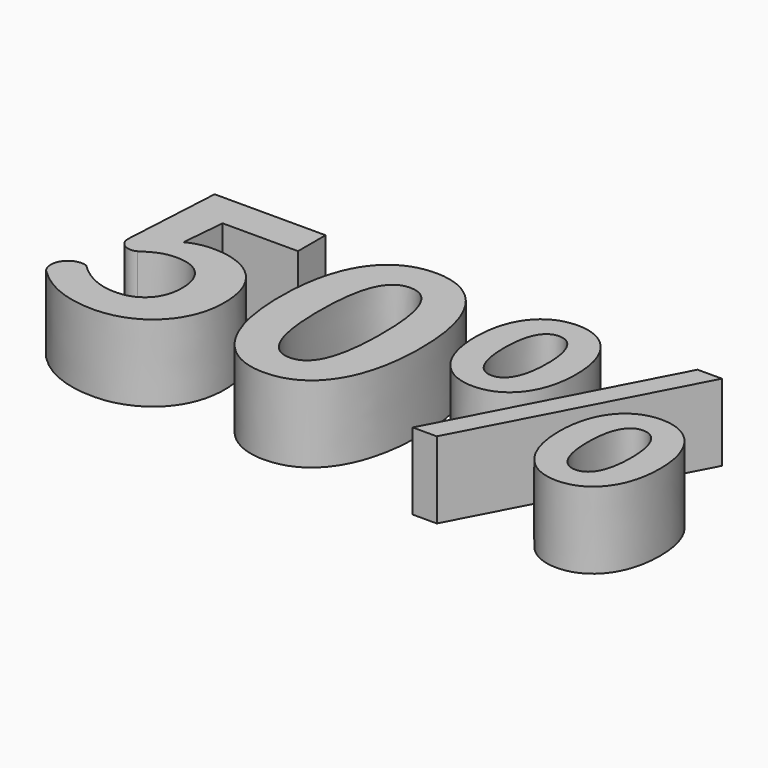
from build123d import *

# Parameters (mm, degrees)
F2_DEPTH = 40


with BuildPart() as f2:
    # F1 (on Top) → F2 (new body)
    with BuildSketch(Plane.XY):
        with BuildLine():
            Line((-37.6012061267, 49.3926707034), (-95.4441113863, 49.3926707034))
            Line((-95.4441113863, 49.3926707034), (-98.3659313836, -3.0631289361))
            ThreePointArc((-98.3659313836, -3.0631289361), (-95.3198653418, -9.0950649064), (-88.5732690488, -9.477436899))
            add(Edge.make_bspline(
                [(-88.5732690488, -9.477436899), (-82.2959213983, -5.3914542465), (-78.780606714, -3.7935839355), (-72.3662987511, -3.7935839355)],
                knots=[0, 0, 0, 0, 1, 1, 1, 1], degree=3))
            add(Edge.make_bspline(
                [(-72.3662987511, -3.7935839355), (-61.4094737612, -3.7935839355), (-54.1049237678, -10.8013865853), (-54.1049237678, -23.3560818864)],
                knots=[0, 0, 0, 0, 1, 1, 1, 1], degree=3))
            add(Edge.make_bspline(
                [(-54.1049237678, -23.3560818864), (-54.1049237678, -36.0705642185), (-61.9801417294, -43.2381538994), (-73.2337140629, -43.2381538994)],
                knots=[0, 0, 0, 0, 1, 1, 1, 1], degree=3))
            add(Edge.make_bspline(
                [(-73.2337140629, -43.2381538994), (-83.3231237411, -43.2381538994), (-90.9244210779, -38.2619292165), (-97.0419816974, -32.2813289094)],
                knots=[0, 0, 0, 0, 1, 1, 1, 1], degree=3))
            ThreePointArc((-97.0419816974, -32.2813289094), (-107.0940288058, -35.4584640814), (-106.9944310633, -46.0001868657))
            add(Edge.make_bspline(
                [(-106.9944310633, -46.0001868657), (-98.9594260706, -54.0351918583), (-87.546066706, -60.7690738834), (-70.4716810966, -60.7690738834)],
                knots=[0, 0, 0, 0, 1, 1, 1, 1], degree=3))
            add(Edge.make_bspline(
                [(-70.4716810966, -60.7690738834), (-50.4526487712, -60.7690738834), (-32.6249814437, -46.8904288961), (-32.6249814437, -22.7854139181)],
                knots=[0, 0, 0, 0, 1, 1, 1, 1], degree=3))
            add(Edge.make_bspline(
                [(-32.6249814437, -22.7854139181), (-32.6249814437, 0.7489330916), (-47.8275761173, 11.5459710505), (-65.9291640695, 11.5459710505)],
                knots=[0, 0, 0, 0, 1, 1, 1, 1], degree=3))
            add(Edge.make_bspline(
                [(-65.9291640695, 11.5459710505), (-70.9053887525, 11.5459710505), (-74.6946240615, 10.5415954264), (-78.9403937451, 8.4871907408)],
                knots=[0, 0, 0, 0, 1, 1, 1, 1], degree=3))
            Line((-78.9403937451, 8.4871907408), (-76.8859890595, 31.4280430636))
            Line((-76.8859890595, 31.4280430636), (-37.6012061267, 31.4280430636))
            Line((-37.6012061267, 31.4280430636), (-37.6012061267, 49.3926707034))
        make_face()
    extrude(amount=F2_DEPTH)


with BuildPart() as f2b:
    # F1 (on Top) → F2, piece 2 (new body)
    with BuildSketch(Plane.XY):
        with BuildLine():
            add(Edge.make_bspline(
                [(54.8926581638, -4.2272915913), (54.8926581638, 33.0259133746), (40.2835581772, 51.4470753891), (18.3699081972, 51.4470753891)],
                knots=[0, 0, 0, 0, 1, 1, 1, 1], degree=3))
            add(Edge.make_bspline(
                [(18.3699081972, 51.4470753891), (-3.6807020952, 51.4470753891), (-18.2898020818, 33.1857004057), (-18.2898020818, -4.2272915913)],
                knots=[0, 0, 0, 0, 1, 1, 1, 1], degree=3))
            add(Edge.make_bspline(
                [(-18.2898020818, -4.2272915913), (-18.2898020818, -41.4804965573), (-3.6807020952, -60.7690738834), (18.3699081972, -60.7690738834)],
                knots=[0, 0, 0, 0, 1, 1, 1, 1], degree=3))
            add(Edge.make_bspline(
                [(18.3699081972, -60.7690738834), (40.2835581772, -60.7690738834), (54.8926581638, -41.4804965573), (54.8926581638, -4.2272915913)],
                knots=[0, 0, 0, 0, 1, 1, 1, 1], degree=3))
        make_face()
        with BuildLine():
            add(Edge.make_bspline(
                [(34.5768784949, -4.2272915913), (34.5768784949, -34.6096542198), (27.569075845, -43.9686088988), (18.3699081972, -43.9686088988)],
                knots=[0, 0, 0, 0, 1, 1, 1, 1], degree=3))
            add(Edge.make_bspline(
                [(18.3699081972, -43.9686088988), (9.0109535183, -43.9686088988), (2.0031508684, -34.6096542198), (2.0031508684, -4.2272915913)],
                knots=[0, 0, 0, 0, 1, 1, 1, 1], degree=3))
            add(Edge.make_bspline(
                [(2.0031508684, -4.2272915913), (2.0031508684, 26.0181107248), (9.0109535183, 34.7835707168), (18.3699081972, 34.7835707168)],
                knots=[0, 0, 0, 0, 1, 1, 1, 1], degree=3))
            add(Edge.make_bspline(
                [(18.3699081972, 34.7835707168), (27.569075845, 34.7835707168), (34.5768784949, 26.0181107248), (34.5768784949, -4.2272915913)],
                knots=[0, 0, 0, 0, 1, 1, 1, 1], degree=3))
        make_face(mode=Mode.SUBTRACT)
    extrude(amount=F2_DEPTH)


with BuildPart() as f2c:
    # F1 (on Top) → F2, piece 3 (new body)
    with BuildSketch(Plane.XY):
        with BuildLine():
            add(Edge.make_bspline(
                [(118.7389904492, 17.3896110452), (118.7389904492, 39.0293404004), (107.7821654593, 51.4470753891), (92.3056501609, 51.4470753891)],
                knots=[0, 0, 0, 0, 1, 1, 1, 1], degree=3))
            add(Edge.make_bspline(
                [(92.3056501609, 51.4470753891), (76.8063081438, 51.4470753891), (66.0092701849, 39.0293404004), (66.0092701849, 17.3896110452)],
                knots=[0, 0, 0, 0, 1, 1, 1, 1], degree=3))
            add(Edge.make_bspline(
                [(66.0092701849, 17.3896110452), (66.0092701849, -4.3642519037), (76.8063081438, -17.0787342358), (92.3056501609, -17.0787342358)],
                knots=[0, 0, 0, 0, 1, 1, 1, 1], degree=3))
            add(Edge.make_bspline(
                [(92.3056501609, -17.0787342358), (107.7821654593, -17.0787342358), (118.7389904492, -4.3642519037), (118.7389904492, 17.3896110452)],
                knots=[0, 0, 0, 0, 1, 1, 1, 1], degree=3))
        make_face()
        with BuildLine():
            add(Edge.make_bspline(
                [(103.5592224944, 17.3896110452), (103.5592224944, 1.479388091), (98.5829978114, -4.9577465907), (92.3056501609, -4.9577465907)],
                knots=[0, 0, 0, 0, 1, 1, 1, 1], degree=3))
            add(Edge.make_bspline(
                [(92.3056501609, -4.9577465907), (86.0283025104, -4.9577465907), (81.1890381398, 1.479388091), (81.1890381398, 17.3896110452)],
                knots=[0, 0, 0, 0, 1, 1, 1, 1], degree=3))
            add(Edge.make_bspline(
                [(81.1890381398, 17.3896110452), (81.1890381398, 33.3226607181), (86.0283025104, 39.3032610251), (92.3056501609, 39.3032610251)],
                knots=[0, 0, 0, 0, 1, 1, 1, 1], degree=3))
            add(Edge.make_bspline(
                [(92.3056501609, 39.3032610251), (98.5829978114, 39.3032610251), (103.5592224944, 33.3226607181), (103.5592224944, 17.3896110452)],
                knots=[0, 0, 0, 0, 1, 1, 1, 1], degree=3))
        make_face(mode=Mode.SUBTRACT)
    extrude(amount=F2_DEPTH)


with BuildPart() as f2d:
    # F1 (on Top) → F2, piece 4 (new body)
    with BuildSketch(Plane.XY):
        Polygon((167.3827280611, 51.4470753891), (154.6910724477, 51.4470753891), (95.9579251576, -60.7690738834), (108.5126204586, -60.7690738834), align=None)
    extrude(amount=F2_DEPTH)


with BuildPart() as f2e:
    # F1 (on Top) → F2, piece 5 (new body)
    with BuildSketch(Plane.XY):
        with BuildLine():
            add(Edge.make_bspline(
                [(170.8980427453, -60.7690738834), (186.2375977313, -60.7690738834), (197.3313830337, -47.8948045202), (197.3313830337, -26.2779018837)],
                knots=[0, 0, 0, 0, 1, 1, 1, 1], degree=3))
            add(Edge.make_bspline(
                [(197.3313830337, -26.2779018837), (197.3313830337, -4.5240389348), (186.2375977313, 7.8936960538), (170.8980427453, 7.8936960538)],
                knots=[0, 0, 0, 0, 1, 1, 1, 1], degree=3))
            add(Edge.make_bspline(
                [(170.8980427453, 7.8936960538), (155.5584877594, 7.8936960538), (144.6016627694, -4.5240389348), (144.6016627694, -26.2779018837)],
                knots=[0, 0, 0, 0, 1, 1, 1, 1], degree=3))
            add(Edge.make_bspline(
                [(144.6016627694, -26.2779018837), (144.6016627694, -47.8948045202), (155.5584877594, -60.7690738834), (170.8980427453, -60.7690738834)],
                knots=[0, 0, 0, 0, 1, 1, 1, 1], degree=3))
        make_face()
        with BuildLine():
            add(Edge.make_bspline(
                [(170.8980427453, -4.2272915913), (177.1753903959, -4.2272915913), (182.1516150788, -10.3676789295), (182.1516150788, -26.2779018837)],
                knots=[0, 0, 0, 0, 1, 1, 1, 1], degree=3))
            add(Edge.make_bspline(
                [(182.1516150788, -26.2779018837), (182.1516150788, -42.2109515566), (177.1753903959, -48.4882992071), (170.8980427453, -48.4882992071)],
                knots=[0, 0, 0, 0, 1, 1, 1, 1], degree=3))
            add(Edge.make_bspline(
                [(170.8980427453, -48.4882992071), (164.6206950948, -48.4882992071), (159.6444704119, -42.2109515566), (159.6444704119, -26.2779018837)],
                knots=[0, 0, 0, 0, 1, 1, 1, 1], degree=3))
            add(Edge.make_bspline(
                [(159.6444704119, -26.2779018837), (159.6444704119, -10.3676789295), (164.6206950948, -4.2272915913), (170.8980427453, -4.2272915913)],
                knots=[0, 0, 0, 0, 1, 1, 1, 1], degree=3))
        make_face(mode=Mode.SUBTRACT)
    extrude(amount=F2_DEPTH)


solid = Compound([f2.part, f2b.part, f2c.part, f2d.part, f2e.part])
